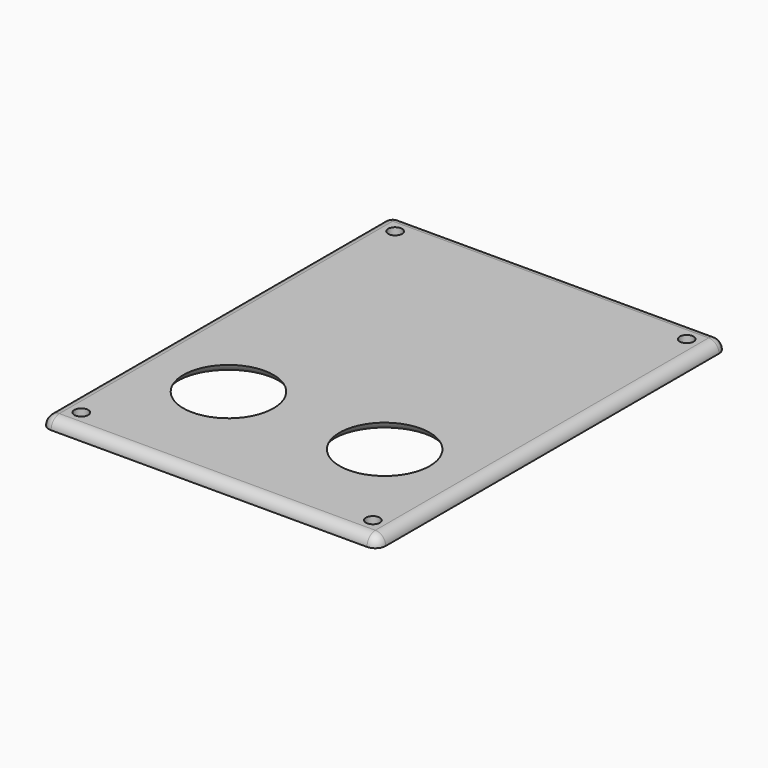
from build123d import *

# Parameters (mm, degrees)
F0_W     = 97
F0_H     = 126
F0_R     = 2
F0_R_2   = 13
F1_DEPTH = 3
F4_R     = 3
F5_R     = 3
F6_R     = 2.99999


# Not quite as in the source:
# - a fillet or chamfer that OpenCascade refuses, or shapes differently, is made with other operations: its cross-section is extruded or revolved along the edge and cut away or added
# - a fillet or chamfer is up to 0.001 mm smaller than in the source, because OpenCascade refuses the exact size


with BuildPart() as f1:
    # F0 (on Top) → F1 (new body)
    with BuildSketch(Plane.XY):
        Rectangle(F0_W, F0_H)
        with Locations((-42, -56.5)):
            Circle(F0_R, mode=Mode.SUBTRACT)
        with Locations((-22.5, -27.884999302)):
            Circle(F0_R_2, mode=Mode.SUBTRACT)
        with Locations((42, -56.5)):
            Circle(F0_R, mode=Mode.SUBTRACT)
        with Locations((22.5, -27.8849992901)):
            Circle(F0_R_2, mode=Mode.SUBTRACT)
        with Locations((-42, 56.5)):
            Circle(F0_R, mode=Mode.SUBTRACT)
        with Locations((42, 56.5)):
            Circle(F0_R, mode=Mode.SUBTRACT)
    extrude(amount=F1_DEPTH)

    # F2: fillet of radius 5 on 1 edges, made by hand

    # F2_s1 → F2_t2 (revolve, cut)
    with BuildSketch(Plane.XZ.offset(27.884999302)):
        with BuildLine():
            ThreePointArc((-9.5, 3), (-7.6560370926, 0.8166998673), (-4.917424305, 0))
            Line((-4.917424305, 0), (-9.5, 0))
            Line((-9.5, 0), (-9.5, 3))
        make_face()
    revolve(axis=Axis((-22.5, -27.884999302, 0), (0, 0, 1)), mode=Mode.SUBTRACT)

    # F3: fillet of radius 5 on 1 edges, made by hand

    # F3_s1 → F3_t2 (revolve, cut)
    with BuildSketch(Plane.XZ.offset(27.8849992901)):
        with BuildLine():
            ThreePointArc((40.082575695, 0), (37.3439629074, 0.8166998673), (35.5, 3))
            Line((35.5, 3), (35.5, 0))
            Line((35.5, 0), (40.082575695, 0))
        make_face()
    revolve(axis=Axis((22.5, -27.8849992901, 0), (0, 0, 1)), mode=Mode.SUBTRACT)

    # F4
    f4_edges = [f1.edges().sort_by_distance(p)[0] for p in [
        (48.5, -63, 1.5),
        (-48.5, -63, 1.5),
    ]]
    fillet(f4_edges, radius=F4_R)

    # F5
    f5_edges = [f1.edges().sort_by_distance(p)[0] for p in [
        (48.5, 63, 1.5),
        (-48.5, 63, 1.5),
    ]]
    fillet(f5_edges, radius=F5_R)

    # F6 (radius 3 in the source; OpenCascade refuses exactly that, so slightly less here)
    f6_edges = [f1.edges().sort_by_distance(p)[0] for p in [
        (0, -63, 3),
        (47.62132, -62.12132, 3),
        (48.5, 0, 3),
        (47.62132, 62.12132, 3),
        (0, 63, 3),
        (-47.62132, 62.12132, 3),
        (-48.5, 0, 3),
        (-47.62132, -62.12132, 3),
    ]]
    fillet(f6_edges, radius=F6_R)


solid = f1.part
